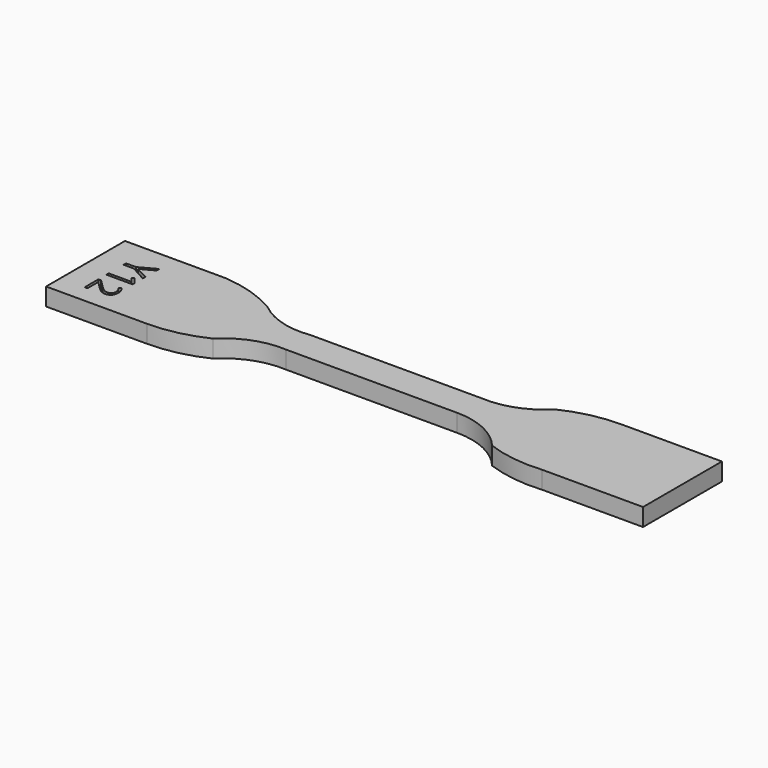
from build123d import *

# Parameters (mm, degrees)
F1_DEPTH     = 3.4
F2_TEXT_SIZE = 7.0564552314
F3_DEPTH     = 1


# Not quite as in the source:
# - Text() gives the source's letters only with a copy of the font that has no kerning and outlines rounded to 1/6400 em; it was checked with that copy


with BuildPart() as f1:
    # F0 (on Top) → F1 (new body)
    with BuildSketch(Plane.XY):
        with BuildLine():
            Line((-14.4320548165, 19.7811394548), (-33.8720548165, 19.7811394548))
            Line((-33.8720548165, 19.7811394548), (-33.8720548165, 0.7811394548))
            Line((-33.8720548165, 0.7811394548), (-14.4320548165, 0.7811394548))
            ThreePointArc((-14.4320548165, 0.7811394548), (-8.9053122052, 1.3996892086), (-3.6520548165, 3.2247301661))
            ThreePointArc((-3.6520548165, 3.2247301661), (1.3014698263, 6.4128780055), (7.1279451835, 7.2811394548))
            Line((7.1279451835, 7.2811394548), (40.1279451835, 7.2811394548))
            ThreePointArc((40.1279451835, 7.2811394548), (46.0837574042, 5.9511158081), (50.9079451835, 2.2137538538))
            ThreePointArc((50.9079451835, 2.2137538538), (56.2191047011, 0.9041953221), (61.6879451835, 0.7811394548))
            Line((61.6879451835, 0.7811394548), (81.1279451835, 0.7811394548))
            Line((81.1279451835, 0.7811394548), (81.1279451835, 19.7811394548))
            Line((81.1279451835, 19.7811394548), (61.6879451835, 19.7811394548))
            ThreePointArc((61.6879451835, 19.7811394548), (56.1612025723, 19.162589701), (50.9079451835, 17.3375487435))
            ThreePointArc((50.9079451835, 17.3375487435), (45.9544205407, 14.1494009041), (40.1279451835, 13.2811394548))
            Line((40.1279451835, 13.2811394548), (7.1279451835, 13.2811394548))
            ThreePointArc((7.1279451835, 13.2811394548), (1.4167452884, 13.6925537245), (-3.6520548165, 16.3560723447))
            ThreePointArc((-3.6520548165, 16.3560723447), (-8.8458057958, 18.686276846), (-14.4320548165, 19.7811394548))
        make_face()
    extrude(amount=F1_DEPTH)

    # F2 (on face) → F3 (cut)
    with BuildSketch(Plane.XY.offset(3.4)):
        with Locations(Location((-29.1824135929, 15.8650862949), (0, 0, -90))):
            Text('Y12', F2_TEXT_SIZE, font='Open Sans', text_align=(TextAlign.LEFT, TextAlign.BOTTOM))
    extrude(amount=-F3_DEPTH, mode=Mode.SUBTRACT)


solid = f1.part
